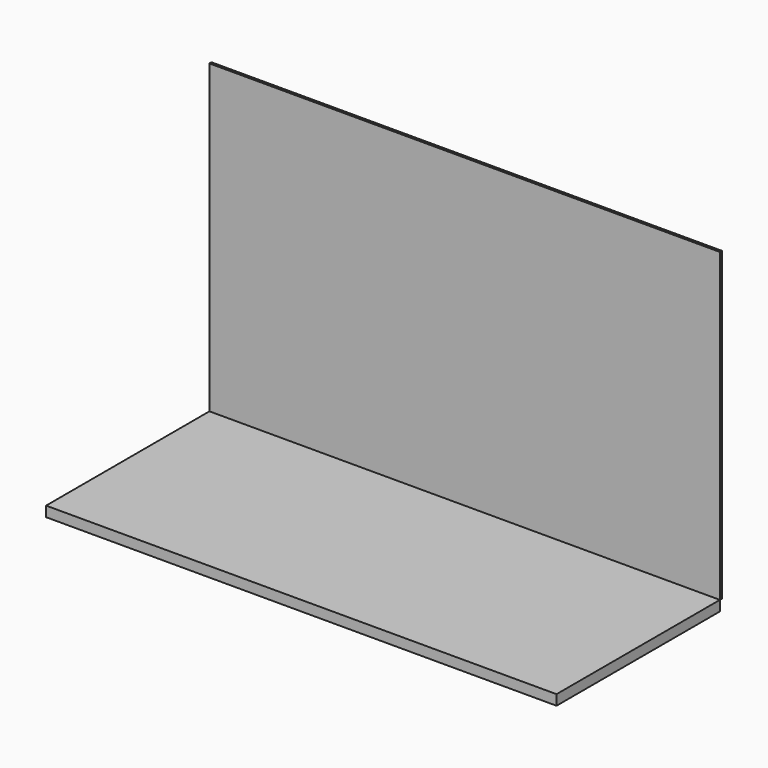
from build123d import *

# Parameters (mm, degrees)
F0_W     = 5000
F0_H     = 2000
F1_DEPTH = 100
F2_W     = 5000
F2_H     = 3000
F3_DEPTH = 25


# Not quite as in the source:
# - the program builds the solid bodies; features that only make, move or delete a surface that nothing else refers to are left out


with BuildPart() as f1:
    # F0 (on Top) → F1 (new body)
    with BuildSketch(Plane.XY):
        with Locations((-2500, -1000)):
            Rectangle(F0_W, F0_H)
    extrude(amount=-F1_DEPTH)


with BuildPart() as f3:
    # F2 (on face) → F3 (new body)
    with BuildSketch(Plane(origin=(0, 0, 0), x_dir=(-1, 0, 0), z_dir=(0, 1, 0))):
        with Locations((2500, 1500)):
            Rectangle(F2_W, F2_H)
    extrude(amount=F3_DEPTH)


solid = Compound([f1.part, f3.part])
